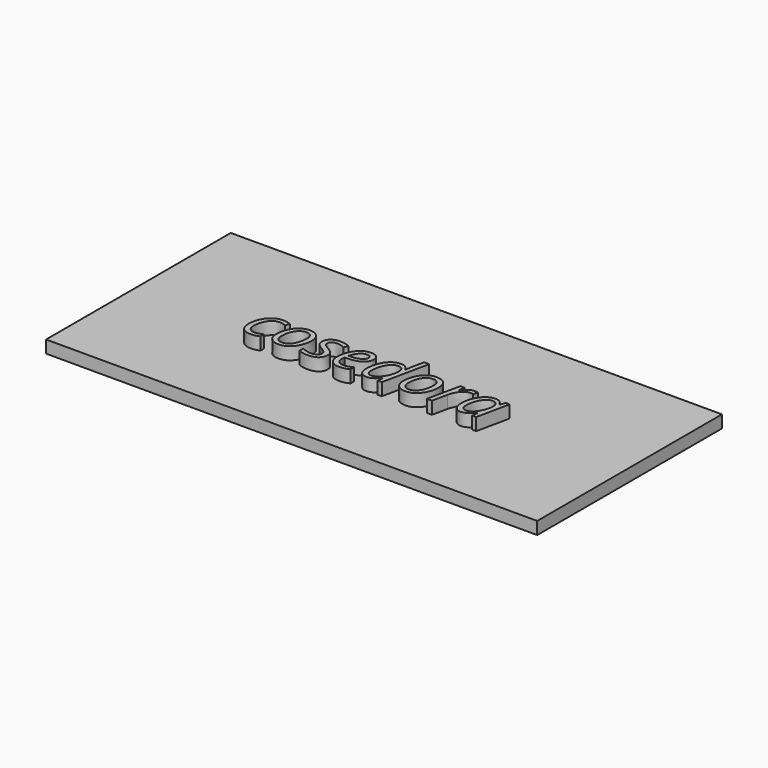
from build123d import *

# Parameters (mm, degrees)
F0_W         = 1000
F0_H         = 470
F1_DEPTH     = 25.4
F2_TEXT_SIZE = 125.4031774507
F3_DEPTH     = 25.4


# Not quite as in the source:
# - Text() gives the source's letters only with a copy of the font that has no kerning and outlines rounded to 1/6400 em; it was checked with that copy


with BuildPart() as f1:
    # F0 (on Top) → F1 (new body)
    with BuildSketch(Plane.XY):
        with Locations((2.158543095, 93.2736457344)):
            Rectangle(F0_W, F0_H)
    extrude(amount=F1_DEPTH)

    # F2 (on face) → F3 (join)
    with BuildSketch(Plane.XY.offset(25.4)):
        with Locations((-255.7343078903, 38.9519208365)):
            Text('cosedora', F2_TEXT_SIZE, font='Open Sans', font_style=FontStyle.ITALIC, text_align=(TextAlign.LEFT, TextAlign.BOTTOM))
    extrude(amount=F3_DEPTH)


solid = f1.part
